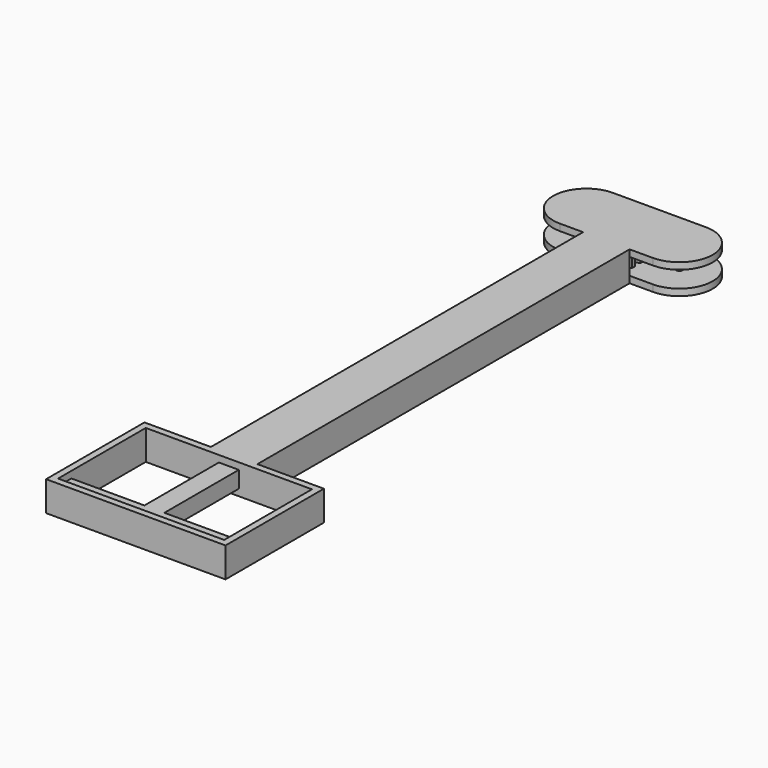
from build123d import *

# Parameters (mm, degrees)
F1_DEPTH      = 5
F3_W          = 50
F3_H          = 5
F4_DEPTH      = 5
F5_W          = 50
F5_H          = 33
F6_DEPTH      = 7
F6_DEPTH_BACK = 2
F9_DEPTH      = 5
F10_W         = 10
F10_H         = 5
F11_DEPTH     = 50
F12_R         = 1
F13_DEPTH     = 5


with BuildPart() as f1:
    # F0 (on Top) → F1 (new body)
    with BuildSketch(Plane.XY):
        Polygon((3, 13), (0, 13), (0, -180), (3, -180), (3, -39.0871235167), (3, -36.9128764833), (3, -35.8871235167), (3, -33.7128764833), (3, -32.6871235167), (3, -30.5128764833), (3, -29.4871235167), (3, -27.3128764833), (3, -26.2871235167), (3, -24.1128764833), (3, -23.0871235167), (3, -20.9128764833), (3, -19.8871235167), (3, -17.7128764833), (3, -16.6871235167), (3, -14.5128764833), (3, -13.4871235167), (3, -11.3128764833), (3, -10.2871235167), (3, -8.1128764833), (3, -7.0871235167), (3, -4.9128764833), (3, -3.8871235167), (3, -1.7128764833), (3, -0.6871235167), (3, 1.4871235167), (3, 2.5128764833), (3, 4.6871235167), (3, 5.7128764833), (3, 7.8871235167), (3, 8.9128764833), (3, 11.0871235167), align=None)
        with BuildLine():
            ThreePointArc((5, 10.5), (4.0421988802, 10.9373096378), (3, 11.0871235167))
            Line((3, 11.0871235167), (3, 8.9128764833))
            ThreePointArc((3, 8.9128764833), (4.0421988802, 9.0626903622), (5, 9.5))
            Line((5, 9.5), (5, 10))
            Line((5, 10), (5, 10.5))
        make_face()
        with BuildLine():
            Line((3, -36.9128764833), (3, -39.0871235167))
            ThreePointArc((3, -39.0871235167), (4.0421988802, -38.9373096378), (5, -38.5))
            Line((5, -38.5), (5, -38))
            Line((5, -38), (5, -37.5))
            ThreePointArc((5, -37.5), (4.0421988802, -37.0626903622), (3, -36.9128764833))
        make_face()
        with BuildLine():
            ThreePointArc((5, 7.3), (4.0421988802, 7.7373096378), (3, 7.8871235167))
            Line((3, 7.8871235167), (3, 5.7128764833))
            ThreePointArc((3, 5.7128764833), (4.0421988802, 5.8626903622), (5, 6.3))
            Line((5, 6.3), (5, 6.8))
            Line((5, 6.8), (5, 7.3))
        make_face()
        with BuildLine():
            Line((3, -33.7128764833), (3, -35.8871235167))
            ThreePointArc((3, -35.8871235167), (4.0421988802, -35.7373096378), (5, -35.3))
            Line((5, -35.3), (5, -34.8))
            Line((5, -34.8), (5, -34.3))
            ThreePointArc((5, -34.3), (4.0421988802, -33.8626903622), (3, -33.7128764833))
        make_face()
        with BuildLine():
            ThreePointArc((5, 4.1), (4.0421988802, 4.5373096378), (3, 4.6871235167))
            Line((3, 4.6871235167), (3, 2.5128764833))
            ThreePointArc((3, 2.5128764833), (4.0421988802, 2.6626903622), (5, 3.1))
            Line((5, 3.1), (5, 3.6))
            Line((5, 3.6), (5, 4.1))
        make_face()
        with BuildLine():
            Line((3, -30.5128764833), (3, -32.6871235167))
            ThreePointArc((3, -32.6871235167), (4.0421988802, -32.5373096378), (5, -32.1))
            Line((5, -32.1), (5, -31.6))
            Line((5, -31.6), (5, -31.1))
            ThreePointArc((5, -31.1), (4.0421988802, -30.6626903622), (3, -30.5128764833))
        make_face()
        with BuildLine():
            ThreePointArc((5, 0.9), (4.0421988802, 1.3373096378), (3, 1.4871235167))
            Line((3, 1.4871235167), (3, -0.6871235167))
            ThreePointArc((3, -0.6871235167), (4.0421988802, -0.5373096378), (5, -0.1))
            Line((5, -0.1), (5, 0.4))
            Line((5, 0.4), (5, 0.9))
        make_face()
        with BuildLine():
            Line((3, -27.3128764833), (3, -29.4871235167))
            ThreePointArc((3, -29.4871235167), (4.0421988802, -29.3373096378), (5, -28.9))
            Line((5, -28.9), (5, -28.4))
            Line((5, -28.4), (5, -27.9))
            ThreePointArc((5, -27.9), (4.0421988802, -27.4626903622), (3, -27.3128764833))
        make_face()
        with BuildLine():
            ThreePointArc((5, -2.3), (4.0421988802, -1.8626903622), (3, -1.7128764833))
            Line((3, -1.7128764833), (3, -3.8871235167))
            ThreePointArc((3, -3.8871235167), (4.0421988802, -3.7373096378), (5, -3.3))
            Line((5, -3.3), (5, -2.8))
            Line((5, -2.8), (5, -2.3))
        make_face()
        with BuildLine():
            Line((3, -24.1128764833), (3, -26.2871235167))
            ThreePointArc((3, -26.2871235167), (4.0421988802, -26.1373096378), (5, -25.7))
            Line((5, -25.7), (5, -25.2))
            Line((5, -25.2), (5, -24.7))
            ThreePointArc((5, -24.7), (4.0421988802, -24.2626903622), (3, -24.1128764833))
        make_face()
        with BuildLine():
            ThreePointArc((5, -5.5), (4.0421988802, -5.0626903622), (3, -4.9128764833))
            Line((3, -4.9128764833), (3, -7.0871235167))
            ThreePointArc((3, -7.0871235167), (4.0421988802, -6.9373096378), (5, -6.5))
            Line((5, -6.5), (5, -6))
            Line((5, -6), (5, -5.5))
        make_face()
        with BuildLine():
            Line((3, -20.9128764833), (3, -23.0871235167))
            ThreePointArc((3, -23.0871235167), (4.0421988802, -22.9373096378), (5, -22.5))
            Line((5, -22.5), (5, -22))
            Line((5, -22), (5, -21.5))
            ThreePointArc((5, -21.5), (4.0421988802, -21.0626903622), (3, -20.9128764833))
        make_face()
        with BuildLine():
            ThreePointArc((5, -8.7), (4.0421988802, -8.2626903622), (3, -8.1128764833))
            Line((3, -8.1128764833), (3, -10.2871235167))
            ThreePointArc((3, -10.2871235167), (4.0421988802, -10.1373096378), (5, -9.7))
            Line((5, -9.7), (5, -9.2))
            Line((5, -9.2), (5, -8.7))
        make_face()
        with BuildLine():
            Line((3, -17.7128764833), (3, -19.8871235167))
            ThreePointArc((3, -19.8871235167), (4.0421988802, -19.7373096378), (5, -19.3))
            Line((5, -19.3), (5, -18.8))
            Line((5, -18.8), (5, -18.3))
            ThreePointArc((5, -18.3), (4.0421988802, -17.8626903622), (3, -17.7128764833))
        make_face()
        with BuildLine():
            ThreePointArc((5, -11.9), (4.0421988802, -11.4626903622), (3, -11.3128764833))
            Line((3, -11.3128764833), (3, -13.4871235167))
            ThreePointArc((3, -13.4871235167), (4.0421988802, -13.3373096378), (5, -12.9))
            Line((5, -12.9), (5, -12.4))
            Line((5, -12.4), (5, -11.9))
        make_face()
        with BuildLine():
            Line((3, -14.5128764833), (3, -16.6871235167))
            ThreePointArc((3, -16.6871235167), (4.0421988802, -16.5373096378), (5, -16.1))
            Line((5, -16.1), (5, -15.6))
            Line((5, -15.6), (5, -15.1))
            ThreePointArc((5, -15.1), (4.0421988802, -14.6626903622), (3, -14.5128764833))
        make_face()
    extrude(amount=F1_DEPTH)

    # F2: F1 across face


with BuildPart() as f1_1:
    add(f1.part)
    add(f1.part.mirror(Plane(origin=(0, -83.5, 2.5), x_dir=(0, -1, 0), z_dir=(-1, 0, 0))))

    # F3 (on face) → F4 (join)
    with BuildSketch(Plane.XZ.offset(180)):
        with Locations((0, 2.5)):
            Rectangle(F3_W, F3_H)
    extrude(amount=F4_DEPTH)


with BuildPart() as f6:
    # F5 (on Top) → F6 (new body, two sides)
    with BuildSketch(Plane.XY) as f6_sk:
        with BuildLine():
            ThreePointArc((14, -10), (21.0710678119, -7.0710678119), (24, 0))
            ThreePointArc((24, 0), (21.0710678119, 7.0710678119), (14, 10))
            ThreePointArc((14, 10), (4, 0), (14, -10))
        make_face()
        with BuildLine():
            ThreePointArc((14, -10), (4, 0), (14, 10))
            Line((14, 10), (0, 10))
            Line((0, 10), (-14, 10))
            ThreePointArc((-14, 10), (-6.9289321881, 7.0710678119), (-4, 0))
            ThreePointArc((-4, 0), (-6.9289321881, -7.0710678119), (-14, -10))
            Line((-14, -10), (-7, -10))
            Line((-7, -10), (-7, -150))
            Line((-7, -150), (-27, -150))
            Line((-27, -150), (-27, -187))
            Line((-27, -187), (0, -187))
            Line((0, -187), (27, -187))
            Line((27, -187), (27, -150))
            Line((27, -150), (7, -150))
            Line((7, -150), (7, -10))
            Line((7, -10), (14, -10))
        make_face()
        with Locations((0, -168.5)):
            Rectangle(F5_W, F5_H, mode=Mode.SUBTRACT)
        with BuildLine():
            ThreePointArc((-4, 0), (-6.9289321881, 7.0710678119), (-14, 10))
            ThreePointArc((-14, 10), (-24, 0), (-14, -10))
            ThreePointArc((-14, -10), (-6.9289321881, -7.0710678119), (-4, 0))
        make_face()
    extrude(amount=F6_DEPTH)
    extrude(f6_sk.sketch, amount=-F6_DEPTH_BACK)

    # F7: cut F1
    add(f1_1.part, mode=Mode.SUBTRACT)

    # F8 (on Top) → F9 (cut)
    with BuildSketch(Plane.XY):
        with BuildLine():
            ThreePointArc((-14, 10), (-24, 0), (-14, -10))
            Line((-14, -10), (14, -10))
            ThreePointArc((14, -10), (24, 0), (14, 10))
            Line((14, 10), (-14, 10))
        make_face()
    extrude(amount=F9_DEPTH, mode=Mode.SUBTRACT)

    # F10 (on face) → F11 (cut)
    with BuildSketch(Plane(origin=(0, -10, 0), x_dir=(-1, 0, 0), z_dir=(0, 1, 0))):
        with Locations((0, 2.5)):
            Rectangle(F10_W, F10_H)
    extrude(amount=-F11_DEPTH, mode=Mode.SUBTRACT)

    # F12 (on Top) → F13 (join, through all)
    with BuildSketch(Plane.XY):
        with Locations((14, 0)):
            Circle(F12_R)
        with Locations((-14, 0)):
            Circle(F12_R)
    extrude(amount=F13_DEPTH)


solid = Compound([f1_1.part, f6.part])
